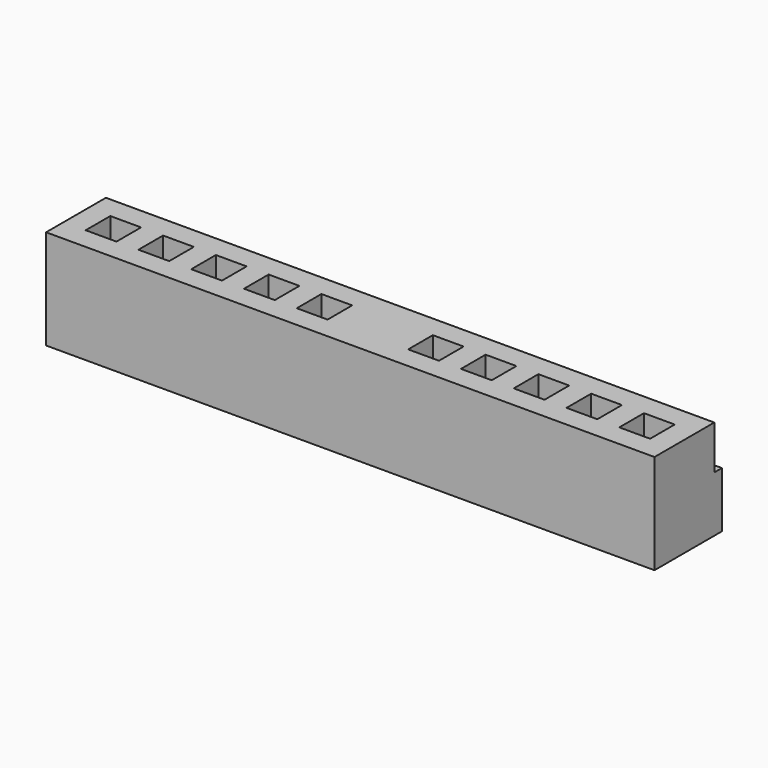
from build123d import *

# Parameters (mm, degrees)
F0_W     = 83
F0_H     = 7.6
F0_W_2   = 78
F0_H_2   = 2.6
F1_DEPTH = 8
F2_W     = 83
F2_H     = 7.6
F2_W_2   = 78
F2_H_2   = 2.6
F3_DEPTH = 3.5
F4_W     = 3
F4_H     = 3
F4_W_2   = 4.2
F4_H_2   = 4.2
F4_W_3   = 11
F5_DEPTH = 6


with BuildPart() as f1:
    # F0 (on Front) → F1 (new body)
    with BuildSketch(Plane.XZ):
        Rectangle(F0_W, F0_H)
        Rectangle(F0_W_2, F0_H_2, mode=Mode.SUBTRACT)
    extrude(amount=F1_DEPTH)

    # F2 (on face) → F3 (join)
    with BuildSketch(Plane.XZ.offset(8)):
        Rectangle(F2_W, F2_H)
        Rectangle(F2_W_2, F2_H_2, mode=Mode.SUBTRACT)
        Rectangle(F2_W_2, F2_H_2)
    extrude(amount=F3_DEPTH)

    # F4 (on face) → F5 (join)
    with BuildSketch(Plane.XY.offset(3.8)):
        with Locations((-40, -10)):
            Rectangle(F4_W, F4_H)
        with Locations((-36.4, -10)):
            Rectangle(F4_W_2, F4_H)
        with Locations((-40, -6.4)):
            Rectangle(F4_W, F4_H_2)
        with Locations((-32.8, -10)):
            Rectangle(F4_W, F4_H)
        with Locations((-40, -2.8)):
            Rectangle(F4_W, F4_H)
        with Locations((-29.2, -10)):
            Rectangle(F4_W_2, F4_H)
        with Locations((-32.8, -6.4)):
            Rectangle(F4_W, F4_H_2)
        with Locations((-36.4, -2.8)):
            Rectangle(F4_W_2, F4_H)
        with Locations((-25.6, -10)):
            Rectangle(F4_W, F4_H)
        with Locations((-32.8, -2.8)):
            Rectangle(F4_W, F4_H)
        with Locations((-22, -10)):
            Rectangle(F4_W_2, F4_H)
        with Locations((-25.6, -6.4)):
            Rectangle(F4_W, F4_H_2)
        with Locations((-29.2, -2.8)):
            Rectangle(F4_W_2, F4_H)
        with Locations((-18.4, -10)):
            Rectangle(F4_W, F4_H)
        with Locations((-25.6, -2.8)):
            Rectangle(F4_W, F4_H)
        with Locations((40, -2.8)):
            Rectangle(F4_W, F4_H)
        with Locations((-14.8, -10)):
            Rectangle(F4_W_2, F4_H)
        with Locations((-18.4, -6.4)):
            Rectangle(F4_W, F4_H_2)
        with Locations((-22, -2.8)):
            Rectangle(F4_W_2, F4_H)
        with Locations((36.4, -2.8)):
            Rectangle(F4_W_2, F4_H)
        with Locations((40, -6.4)):
            Rectangle(F4_W, F4_H_2)
        with Locations((-11.2, -10)):
            Rectangle(F4_W, F4_H)
        with Locations((-18.4, -2.8)):
            Rectangle(F4_W, F4_H)
        with Locations((32.8, -2.8)):
            Rectangle(F4_W, F4_H)
        with Locations((40, -10)):
            Rectangle(F4_W, F4_H)
        with Locations((-7.6, -10)):
            Rectangle(F4_W_2, F4_H)
        with Locations((-11.2, -6.4)):
            Rectangle(F4_W, F4_H_2)
        with Locations((-14.8, -2.8)):
            Rectangle(F4_W_2, F4_H)
        with Locations((29.2, -2.8)):
            Rectangle(F4_W_2, F4_H)
        with Locations((32.8, -6.4)):
            Rectangle(F4_W, F4_H_2)
        with Locations((36.4, -10)):
            Rectangle(F4_W_2, F4_H)
        with Locations((0, -10)):
            Rectangle(F4_W_3, F4_H)
        with Locations((-11.2, -2.8)):
            Rectangle(F4_W, F4_H)
        with Locations((25.6, -2.8)):
            Rectangle(F4_W, F4_H)
        with Locations((32.8, -10)):
            Rectangle(F4_W, F4_H)
        with Locations((7.6, -10)):
            Rectangle(F4_W_2, F4_H)
        with Locations((0, -6.4)):
            Rectangle(F4_W_3, F4_H_2)
        with Locations((-7.6, -2.8)):
            Rectangle(F4_W_2, F4_H)
        with Locations((22, -2.8)):
            Rectangle(F4_W_2, F4_H)
        with Locations((25.6, -6.4)):
            Rectangle(F4_W, F4_H_2)
        with Locations((29.2, -10)):
            Rectangle(F4_W_2, F4_H)
        with Locations((11.2, -10)):
            Rectangle(F4_W, F4_H)
        with Locations((0, -2.8)):
            Rectangle(F4_W_3, F4_H)
        with Locations((18.4, -2.8)):
            Rectangle(F4_W, F4_H)
        with Locations((25.6, -10)):
            Rectangle(F4_W, F4_H)
        with Locations((14.8, -10)):
            Rectangle(F4_W_2, F4_H)
        with Locations((11.2, -6.4)):
            Rectangle(F4_W, F4_H_2)
        with Locations((7.6, -2.8)):
            Rectangle(F4_W_2, F4_H)
        with Locations((14.8, -2.8)):
            Rectangle(F4_W_2, F4_H)
        with Locations((18.4, -6.4)):
            Rectangle(F4_W, F4_H_2)
        with Locations((22, -10)):
            Rectangle(F4_W_2, F4_H)
        with Locations((18.4, -10)):
            Rectangle(F4_W, F4_H)
        with Locations((11.2, -2.8)):
            Rectangle(F4_W, F4_H)
    extrude(amount=F5_DEPTH)


solid = f1.part
